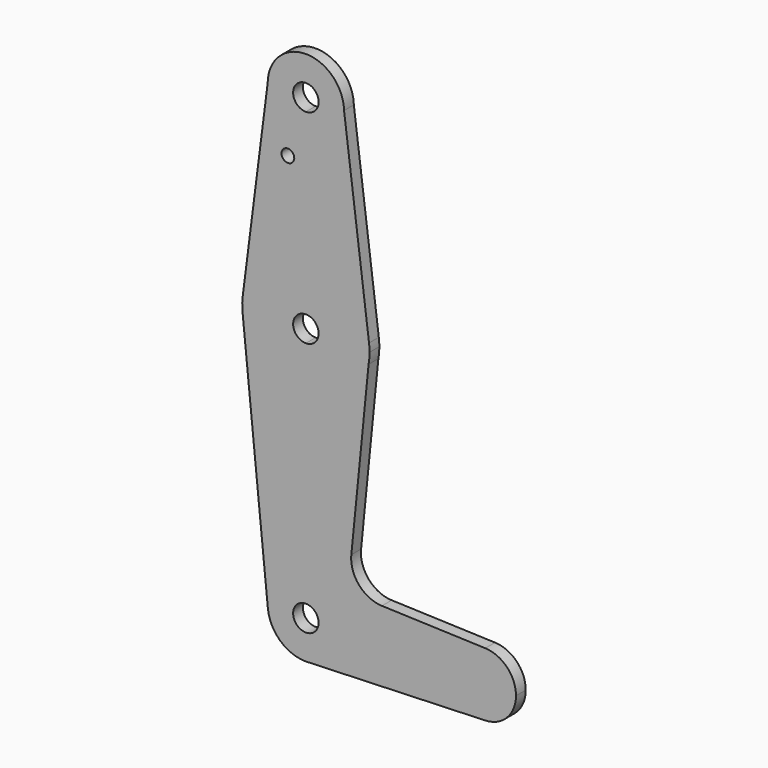
from build123d import *

# Parameters (mm, degrees)
F0_R     = 1.5875
F1_DEPTH = 3.048


# Not quite as in the source:
# - ends of sketch curves that miss each other by under 0.0002 mm in the source are joined


with BuildPart() as f1:
    # F0 (on Front) → F1 (new body)
    with BuildSketch(Plane.XZ):
        with BuildLine():
            ThreePointArc((15.6424620156, -2.7072138984), (15.8167586676, -1.3585912746), (15.875, 0))
            ThreePointArc((15.875, 0), (15.8431224716, 1.0055323711), (15.7476179088, 2.0070264572))
            ThreePointArc((15.7476179088, 2.0070264572), (10.4917605766, 11.9137980931), (0, 15.875))
            Line((0, 15.875), (0, 3.175))
            ThreePointArc((0, 3.175), (2.2450640303, 2.2450640303), (3.175, 0))
            ThreePointArc((3.175, 0), (2.2450640303, -2.2450640303), (0, -3.175))
            Line((0, -3.175), (0, -15.875))
            ThreePointArc((0, -15.875), (10.2234682071, -12.1448064134), (15.6424620156, -2.7072138984))
        make_face()
        with BuildLine():
            ThreePointArc((0, 15.875), (10.4917605766, 11.9137980931), (15.7476179088, 2.0070264572))
            Line((15.7476179088, 2.0070264572), (9.5227233065, 51.0082446367))
            ThreePointArc((9.5227233065, 51.0082446367), (9.5244308096, 50.9041285408), (9.525, 50.8))
            ThreePointArc((9.525, 50.8), (6.7351920908, 44.0648079092), (0, 41.275))
            Line((0, 41.275), (0, 15.875))
        make_face()
        with BuildLine():
            Line((11.3282274792, -45.9148055684), (15.6424620156, -2.7072138984))
            ThreePointArc((15.6424620156, -2.7072138984), (10.2234682071, -12.1448064134), (0, -15.875))
            Line((0, -15.875), (0, -53.975))
            ThreePointArc((0, -53.975), (6.7351920908, -56.7648079092), (9.525, -63.5))
            Line((9.525, -63.5), (36.5125, -63.5))
            ThreePointArc((36.5125, -63.5), (38.9380895153, -57.7883672161), (44.7324052746, -55.5675253854))
            Line((44.7324052746, -55.5675253854), (18.9562332139, -54.6498638357))
            ThreePointArc((18.9562332139, -54.6498638357), (13.2508040617, -51.9340478454), (11.3282274792, -45.9148055684))
        make_face()
        with BuildLine():
            Line((0, 3.175), (0, 15.875))
            ThreePointArc((0, 15.875), (-10.4917605136, 11.9137981486), (-15.7476178875, 2.0070266238))
            ThreePointArc((-15.7476178875, 2.0070266238), (-15.874347828, -0.1438959179), (-15.7086470576, -2.2921676682))
            ThreePointArc((-15.7086470576, -2.2921676682), (-10.383339137, -12.0084092771), (0, -15.875))
            Line((0, -15.875), (0, -3.175))
            ThreePointArc((0, -3.175), (-3.175, 0), (0, 3.175))
        make_face()
        with BuildLine():
            ThreePointArc((-15.7476178875, 2.0070266238), (-10.4917605136, 11.9137981486), (0, 15.875))
            Line((0, 15.875), (0, 41.275))
            ThreePointArc((0, 41.275), (-6.7463579351, 44.0759922954), (-9.5249475556, 50.8316079556))
            Line((-9.5249475556, 50.8316079556), (-15.7476178875, 2.0070266238))
        make_face()
        with Locations((-4.4804564677, 36.5252)):
            Circle(F0_R, mode=Mode.SUBTRACT)
        with BuildLine():
            ThreePointArc((9.525, 50.8), (9.5244308096, 50.9041285408), (9.5227233065, 51.0082446367))
            ThreePointArc((9.5227233065, 51.0082446367), (-0.0883253423, 60.3245904707), (-9.5249475556, 50.8316079556))
            ThreePointArc((-9.5249475556, 50.8316079556), (-6.7463579351, 44.0759922954), (0, 41.275))
            ThreePointArc((0, 41.275), (6.7351920908, 44.0648079092), (9.525, 50.8))
        make_face()
        with BuildLine():
            ThreePointArc((3.175, 50.8), (2.2450640303, 48.5549359697), (0, 47.625))
            ThreePointArc((0, 47.625), (-2.2450640303, 53.0450640303), (3.175, 50.8))
        make_face(mode=Mode.SUBTRACT)
        with BuildLine():
            Line((0, -53.975), (0, -15.875))
            ThreePointArc((0, -15.875), (-10.383339137, -12.0084092771), (-15.7086470576, -2.2921676682))
            Line((-15.7086470576, -2.2921676682), (-9.4774971077, -64.4500913501))
            ThreePointArc((-9.4774971077, -64.4500913501), (-7.0631170566, -57.1095381665), (0, -53.975))
        make_face()
        with BuildLine():
            Line((0, -60.325), (0, -53.975))
            ThreePointArc((0, -53.975), (-7.0631170566, -57.1095381665), (-9.4774971077, -64.4500913501))
            ThreePointArc((-9.4774971077, -64.4500913501), (-6.3904618335, -70.5631170566), (0, -73.025))
            Line((0, -73.025), (0.6773435479, -73.000885786))
            ThreePointArc((0.6773435479, -73.000885786), (6.9705567315, -69.9912990883), (9.525, -63.5))
            Line((9.525, -63.5), (3.175, -63.5))
            ThreePointArc((3.175, -63.5), (-2.2450640303, -65.7450640303), (0, -60.325))
        make_face()
        with BuildLine():
            Line((36.5125, -63.5), (9.525, -63.5))
            ThreePointArc((9.525, -63.5), (6.9705567315, -69.9912990883), (0.6773435479, -73.000885786))
            Line((0.6773435479, -73.000885786), (44.7324052746, -71.4324746146))
            ThreePointArc((44.7324052746, -71.4324746146), (38.9380895153, -69.2116327839), (36.5125, -63.5))
        make_face()
        with BuildLine():
            ThreePointArc((52.3875, -63.5), (50.1616327839, -57.9880895153), (44.7324052746, -55.5675253854))
            ThreePointArc((44.7324052746, -55.5675253854), (38.9380895153, -57.7883672161), (36.5125, -63.5))
            ThreePointArc((36.5125, -63.5), (38.9380895153, -69.2116327839), (44.7324052746, -71.4324746146))
            ThreePointArc((44.7324052746, -71.4324746146), (50.1616327839, -69.0119104847), (52.3875, -63.5))
        make_face()
        with BuildLine():
            Line((0.6773435479, -73.000885786), (0, -73.025))
            ThreePointArc((0, -73.025), (0.3388863295, -73.0189695375), (0.6773435479, -73.000885786))
        make_face()
        with BuildLine():
            ThreePointArc((9.525, -63.5), (6.7351920908, -56.7648079092), (0, -53.975))
            Line((0, -53.975), (0, -60.325))
            ThreePointArc((0, -60.325), (2.2450640303, -61.2549359697), (3.175, -63.5))
            Line((3.175, -63.5), (9.525, -63.5))
        make_face()
    extrude(amount=F1_DEPTH)


solid = f1.part
